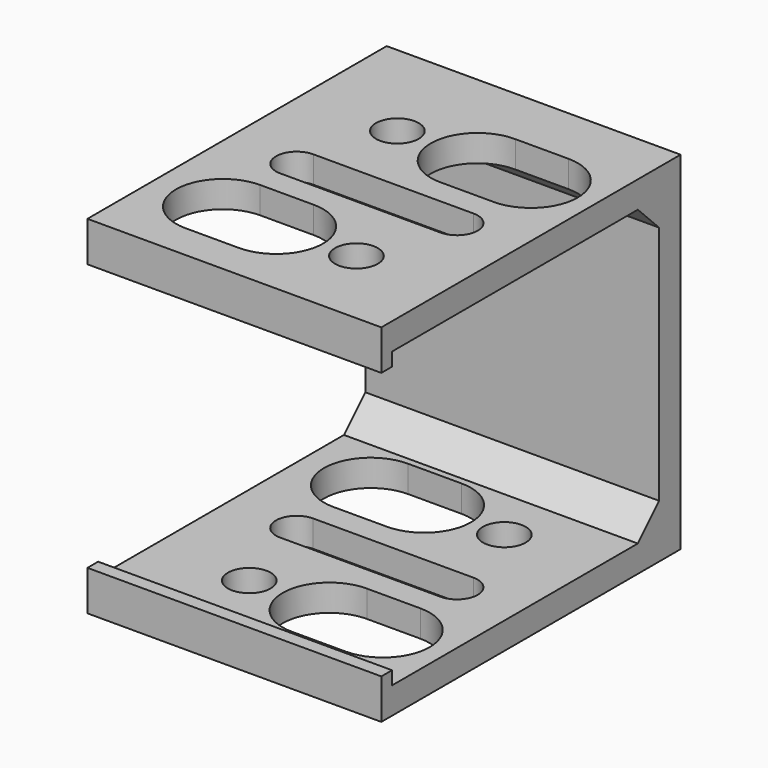
from build123d import *

# Parameters (mm, degrees)
F1_DEPTH  = 27.94
F2_R      = 2.032
F3_DEPTH  = 2.54
F4_R      = 2.032
F5_DEPTH  = 2.54
F6_SIZE   = 2.54
F7_W      = 27.94
F7_H      = 1.27
F8_DEPTH  = 1.27
F9_W      = 27.94
F9_H      = 1.27
F10_DEPTH = 1.27


with BuildPart() as f1:
    # F0 (on Right) → F1 (new body)
    with BuildSketch(Plane.YZ):
        Polygon((0, 30.226001516), (-35.56, 30.226001516), (-35.56, 27.686001516), (-2.54, 27.686001516), (-2.54, -0.253998484), (-35.56, -0.253998484), (-35.56, -2.793998484), (0, -2.793998484), align=None)
    extrude(amount=F1_DEPTH)

    # F2 (on face) → F3 (cut, through all)
    with BuildSketch(Plane.XY.offset(30.226001516)):
        with Locations((9.144, -10.16)):
            Circle(F2_R)
        with Locations((19.3227036137, -27.7468244076)):
            Circle(F2_R)
        with BuildLine():
            Line((21.8533518069, -16.9894844152), (6.6133518069, -16.9894844152))
            ThreePointArc((6.6133518069, -16.9894844152), (4.6494240183, -18.9534122038), (6.6133518069, -20.9173399924))
            Line((6.6133518069, -20.9173399924), (21.8533518069, -20.9173399924))
            ThreePointArc((21.8533518069, -20.9173399924), (23.8172795954, -18.9534122038), (21.8533518069, -16.9894844152))
        make_face()
        with BuildLine():
            ThreePointArc((21.8439999996, -14.605), (26.2890393498, -10.1786250789), (21.8814072278, -5.715))
            Line((21.8814072278, -5.715), (16.8014072278, -5.715))
            ThreePointArc((16.8014072278, -5.715), (12.3189606494, -10.1412175195), (16.7639999996, -14.605))
            Line((16.7639999996, -14.605), (21.8439999996, -14.605))
        make_face()
        with BuildLine():
            ThreePointArc((11.7027036137, -32.1918244076), (16.1477036137, -27.7468244076), (11.7027036137, -23.3018244076))
            Line((11.7027036137, -23.3018244076), (6.6227036137, -23.3018244076))
            ThreePointArc((6.6227036137, -23.3018244076), (2.1777036137, -27.7468244076), (6.6227036137, -32.1918244076))
            Line((6.6227036137, -32.1918244076), (11.7027036137, -32.1918244076))
        make_face()
    extrude(amount=-F3_DEPTH, mode=Mode.SUBTRACT)

    # F4 (on face) → F5 (cut, through all)
    with BuildSketch(Plane(origin=(0, 0, -2.793998484), x_dir=(1, 0, 0), z_dir=(0, 0, -1))):
        with Locations((9.1366654938, 27.746792541)):
            Circle(F4_R)
        with Locations((19.3154241667, 10.16)):
            Circle(F4_R)
        with BuildLine():
            Line((21.8460448303, 20.9173240591), (6.6060448303, 20.9173240591))
            ThreePointArc((6.6060448303, 20.9173240591), (4.6421170417, 18.9533962705), (6.6060448303, 16.9894684819))
            Line((6.6060448303, 16.9894684819), (21.8460448303, 16.9894684819))
            ThreePointArc((21.8460448303, 16.9894684819), (23.8099726188, 18.9533962705), (21.8460448303, 20.9173240591))
        make_face()
        with BuildLine():
            ThreePointArc((21.8356585741, 23.3013725448), (26.2811203019, 27.7276136907), (21.8741828399, 32.1922125373))
            Line((21.8741828399, 32.1922125373), (16.7951897592, 32.1922125373))
            ThreePointArc((16.7951897592, 32.1922125373), (12.3112037656, 27.7661383181), (16.7566654934, 23.3013725448))
            Line((16.7566654934, 23.3013725448), (21.8356585741, 23.3013725448))
        make_face()
        with BuildLine():
            ThreePointArc((11.6954241667, 5.715), (16.1404241667, 10.16), (11.6954241667, 14.605))
            Line((11.6954241667, 14.605), (6.6154241667, 14.605))
            ThreePointArc((6.6154241667, 14.605), (2.1704241667, 10.16), (6.6154241667, 5.715))
            Line((6.6154241667, 5.715), (11.6954241667, 5.715))
        make_face()
    extrude(amount=-F5_DEPTH, mode=Mode.SUBTRACT)

    # F6
    f6_edges = [f1.edges().sort_by_distance(p)[0] for p in [
        (13.97, -2.54, -0.253998),
        (13.97, -2.54, 27.686002),
    ]]
    chamfer(f6_edges, length=F6_SIZE)

    # F7 (on face) → F8 (join)
    with BuildSketch(Plane.XY.offset(-0.253998484)):
        with Locations((13.97, -34.925)):
            Rectangle(F7_W, F7_H)
    extrude(amount=F8_DEPTH)

    # F9 (on face) → F10 (join)
    with BuildSketch(Plane(origin=(0, 0, 27.686001516), x_dir=(1, 0, 0), z_dir=(0, 0, -1))):
        with Locations((13.97, 34.925)):
            Rectangle(F9_W, F9_H)
    extrude(amount=F10_DEPTH)


solid = f1.part
